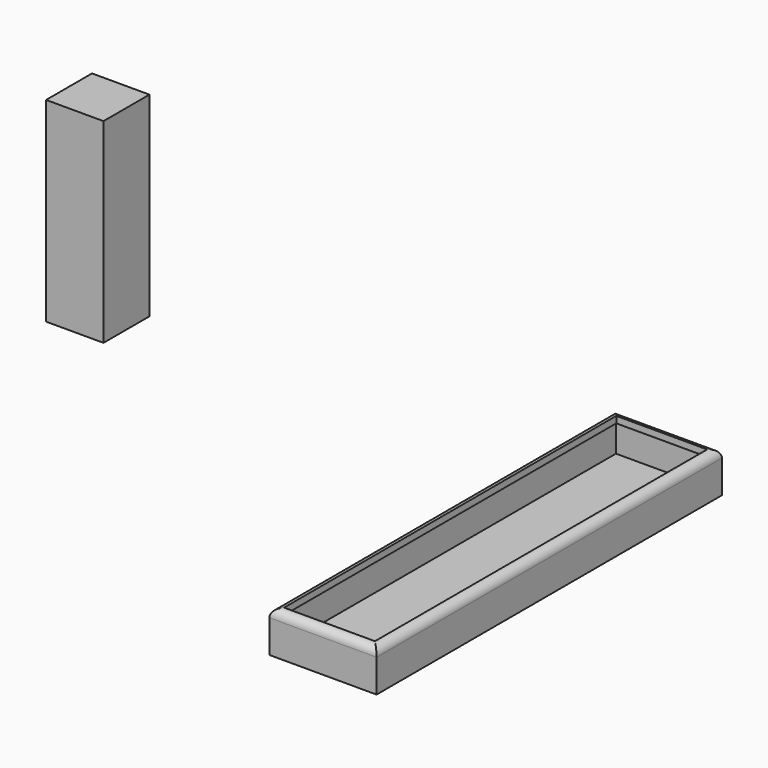
from build123d import *

# Parameters (mm, degrees)
F0_W     = 65.4036104679
F0_H     = 263.1338536739
F1_DEPTH = 25
F2_R     = 5
F3_T     = -4
F4_W     = 35
F4_H     = 35
F5_DEPTH = 119


# Not quite as in the source:
# - a shell that OpenCascade refuses in one call is made with other operations: the cavity is built on its own and cut out


with BuildPart() as f1:
    # F0 (on Top) → F1 (new body)
    with BuildSketch(Plane.XY):
        with Locations((-151.4164656401, -58.0413490534)):
            Rectangle(F0_W, F0_H)
    extrude(amount=F1_DEPTH)

    # F2
    f2_edges = [f1.edges().sort_by_distance(p)[0] for p in [
        (-184.118271, -58.041349, 25),
        (-151.416466, -189.608276, 25),
        (-118.71466, -58.041349, 25),
        (-151.416466, 73.525578, 25),
    ]]
    fillet(f2_edges, radius=F2_R)

    # F3: a shell. OpenCascade refuses it in one call, so the cavity is built on its own and cut out:
    # the body offset inwards by the wall thickness, plus a prism from it out through each open face.
    f3_core = offset(f1.part, amount=F3_T, mode=Mode.PRIVATE)
    f3_exits = [f3_core.faces().sort_by_distance(p)[0] for p in [
        (-151.416466, -58.041349, 21),
    ]]
    add(f3_core, mode=Mode.SUBTRACT)
    extrude(f3_exits, amount=-F3_T, mode=Mode.SUBTRACT)


with BuildPart() as f5:
    # F4 (on Top) → F5 (new body)
    with BuildSketch(Plane.XY):
        with Locations((-464.2132538557, 29.8084301734)):
            Rectangle(F4_W, F4_H)
    extrude(amount=F5_DEPTH)


solid = Compound([f1.part, f5.part])
